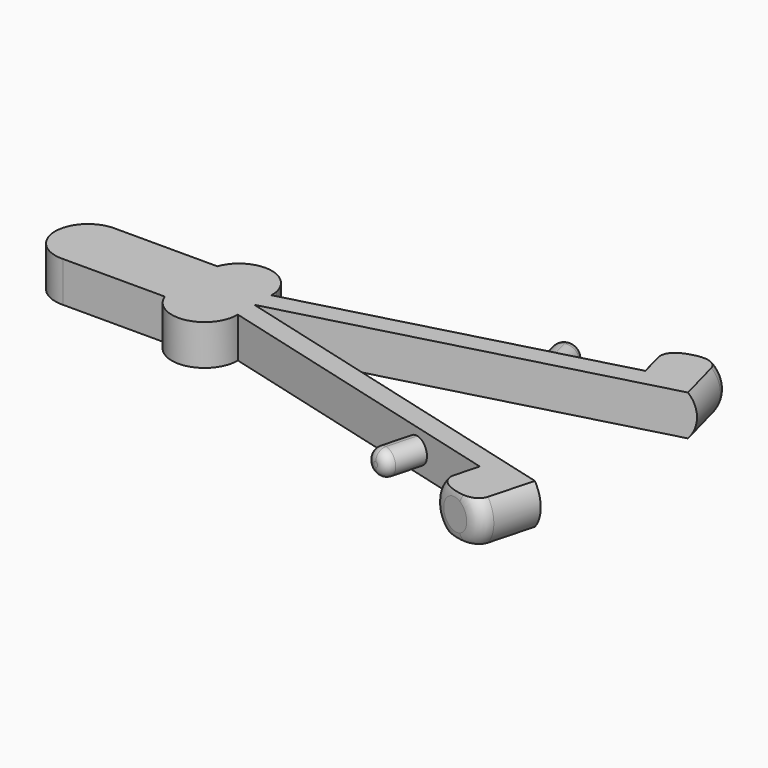
from build123d import *

# Parameters (mm, degrees)
F1_DEPTH    = 8
F4_DEPTH    = 12
F5_DEPTH    = 12
F6_DEPTH    = 4
F7_T2_ANGLE = 226.9097490639
F7_T4_ANGLE = 226.9097490639
F8_R        = 2


# Not quite as in the source:
# - a fillet or chamfer that OpenCascade refuses, or shapes differently, is made with other operations: its cross-section is extruded or revolved along the edge and cut away or added
# - a feature names something its author has since deleted; it is built from what else it names


with BuildPart() as f1:
    # F0 (on Top) → F1 (new body)
    with BuildSketch(Plane.XY):
        with BuildLine():
            ThreePointArc((-26.2934756426, -6.4967182246), (-21.8313594954, -4.5225872947), (-20, 0))
            ThreePointArc((-20, 0), (-21.8313594954, 4.5225872947), (-26.2934756426, 6.4967182246))
            ThreePointArc((-26.2934756426, 6.4967182246), (-33, 0), (-26.2934756426, -6.4967182246))
        make_face()
        with BuildLine():
            ThreePointArc((4.9180788932, 0), (0, 2.25), (-4.9180788932, 0))
            ThreePointArc((-4.9180788932, 0), (0, -2.25), (4.9180788932, 0))
        make_face()
        with BuildLine():
            Line((6.4380174247, 0), (6.3926786471, 3.0737093407))
            ThreePointArc((6.3926786471, 3.0737093407), (5.8604804677, 1.4384579519), (4.9180788932, 0))
            ThreePointArc((4.9180788932, 0), (6.0748085227, -1.9377064606), (6.4992929884, -4.1541321195))
            Line((6.4992929884, -4.1541321195), (6.4380174247, 0))
        make_face()
        with BuildLine():
            ThreePointArc((-26.2934756426, 6.4967182246), (-21.8313594954, 4.5225872947), (-20, 0))
            ThreePointArc((-20, 0), (-21.8313594954, -4.5225872947), (-26.2934756426, -6.4967182246))
            Line((-26.2934756426, -6.4967182246), (-6.0993653128, -6.4967182246))
            ThreePointArc((-6.0993653128, -6.4967182246), (-6.3951431673, -3.0871827877), (-4.9180788932, 0))
            ThreePointArc((-4.9180788932, 0), (-6.3951431673, 3.0871827877), (-6.0993653128, 6.4967182246))
            Line((-6.0993653128, 6.4967182246), (-26.2934756426, 6.4967182246))
        make_face()
        with BuildLine():
            ThreePointArc((-4.9180788932, 0), (-6.3951431673, -3.0871827877), (-6.0993653128, -6.4967182246))
            ThreePointArc((-6.0993653128, -6.4967182246), (1.141079635, -10.6490575296), (6.5, -4.25))
            ThreePointArc((6.5, -4.25), (6.4998232447, -4.2020647563), (6.4992929884, -4.1541321195))
            ThreePointArc((6.4992929884, -4.1541321195), (6.0748085227, -1.9377064606), (4.9180788932, 0))
            ThreePointArc((4.9180788932, 0), (0, -2.25), (-4.9180788932, 0))
        make_face()
        with BuildLine():
            ThreePointArc((6.3552032224, 5.614328407), (0.4593650036, 10.7337476658), (-6.0993653128, 6.4967182246))
            ThreePointArc((-6.0993653128, 6.4967182246), (-6.3951431673, 3.0871827877), (-4.9180788932, 0))
            ThreePointArc((-4.9180788932, 0), (0, 2.25), (4.9180788932, 0))
            ThreePointArc((4.9180788932, 0), (5.8604804677, 1.4384579519), (6.3926786471, 3.0737093407))
            Line((6.3926786471, 3.0737093407), (6.3552032224, 5.614328407))
        make_face()
        with BuildLine():
            ThreePointArc((6.5, 4.25), (6.4636994417, 4.9359952822), (6.3552032224, 5.614328407))
            Line((6.3552032224, 5.614328407), (6.3926786471, 3.0737093407))
            ThreePointArc((6.3926786471, 3.0737093407), (6.4731140576, 3.6594118212), (6.5, 4.25))
        make_face()
    extrude(amount=F1_DEPTH)



with BuildPart() as f4:
    # F3 (on line) → F4 (new body)
    with BuildSketch(Plane(origin=(0.4312653925, -1.6095043562, 0), x_dir=(-0.9659258263, -0.2588190451, 0), z_dir=(-0.2588190451, 0.9659258263, 0))):
        with BuildLine():
            Line((-79.4407832557, 0), (-74.9686473007, 0))
            Line((-74.9686473007, 0), (-74.9686473007, 8))
            Line((-74.9686473007, 8), (-79.4407832557, 8))
            ThreePointArc((-79.4407832557, 8), (-80.9686473007, 4), (-79.4407832557, 0))
        make_face()
        with BuildLine():
            Line((-74.9686473007, 8), (-74.9686473007, 0))
            Line((-74.9686473007, 0), (-70.4965113457, 0))
            ThreePointArc((-70.4965113457, 0), (-69.3636131469, 1.8590674614), (-68.9686473007, 4))
            ThreePointArc((-68.9686473007, 4), (-69.3636131469, 6.1409325386), (-70.4965113457, 8))
            Line((-70.4965113457, 8), (-74.9686473007, 8))
        make_face()
    extrude(amount=F4_DEPTH)


with BuildPart() as f5:
    # F3 (on line) → F5 (new body)
    with BuildSketch(Plane(origin=(0.4312653925, -1.6095043562, 0), x_dir=(-0.9659258263, -0.2588190451, 0), z_dir=(-0.2588190451, 0.9659258263, 0))):
        with BuildLine():
            ThreePointArc((-54.2186473007, 6.5), (-56.7186473007, 4), (-54.2186473007, 1.5))
            Line((-54.2186473007, 1.5), (-54.2186473007, 4))
            Line((-54.2186473007, 4), (-54.2186473007, 6.5))
        make_face()
        with BuildLine():
            ThreePointArc((-51.7186473007, 4), (-52.4508803477, 5.767766953), (-54.2186473007, 6.5))
            Line((-54.2186473007, 6.5), (-54.2186473007, 4))
            Line((-54.2186473007, 4), (-51.7186473007, 4))
        make_face()
        with BuildLine():
            Line((-54.2186473007, 4), (-54.2186473007, 1.5))
            ThreePointArc((-54.2186473007, 1.5), (-52.4508803477, 2.232233047), (-51.7186473007, 4))
            Line((-51.7186473007, 4), (-54.2186473007, 4))
        make_face()
    extrude(amount=F5_DEPTH)


with BuildPart() as f1_1:
    add(f1.part)

    add(f4.part)  # F6 merges F4

    add(f5.part)  # F6 merges F5
    # F3 (on line) → F6 (join)
    with BuildSketch(Plane(origin=(0.4312653925, -1.6095043562, 0), x_dir=(-0.9659258263, -0.2588190451, 0), z_dir=(-0.2588190451, 0.9659258263, 0))):
        with BuildLine():
            Line((-54.2186473007, 1.5), (-54.2186473007, 0))
            Line((-54.2186473007, 0), (-6.2186473007, 0))
            Line((-6.2186473007, 0), (-6.2186473007, 4))
            Line((-6.2186473007, 4), (-51.7186473007, 4))
            ThreePointArc((-51.7186473007, 4), (-52.4508803477, 2.232233047), (-54.2186473007, 1.5))
        make_face()
        with BuildLine():
            Line((-6.2186473007, 8), (-54.2186473007, 8))
            Line((-54.2186473007, 8), (-54.2186473007, 6.5))
            ThreePointArc((-54.2186473007, 6.5), (-52.4508803477, 5.767766953), (-51.7186473007, 4))
            Line((-51.7186473007, 4), (-6.2186473007, 4))
            Line((-6.2186473007, 4), (-6.2186473007, 8))
        make_face()
        with BuildLine():
            ThreePointArc((-68.9686473007, 4), (-69.3636131469, 1.8590674614), (-70.4965113457, 0))
            Line((-70.4965113457, 0), (-54.2186473007, 0))
            Line((-54.2186473007, 0), (-54.2186473007, 1.5))
            ThreePointArc((-54.2186473007, 1.5), (-56.7186473007, 4), (-54.2186473007, 6.5))
            Line((-54.2186473007, 6.5), (-54.2186473007, 8))
            Line((-54.2186473007, 8), (-70.4965113457, 8))
            ThreePointArc((-70.4965113457, 8), (-69.3636131469, 6.1409325386), (-68.9686473007, 4))
        make_face()
    extrude(amount=F6_DEPTH)

    # F7: fillet of radius 3 on 2 edges, made by hand

    # F7_s1 → F7_t2 (revolve, cut)
    with BuildSketch(Plane(origin=(62.3527130216, 16.7073591, 28.0076976241), x_dir=(-0.2588190451, 0.9659258263, 0), z_dir=(0.8861150843, 0.2374338212, 0.3980266798))):
        with BuildLine():
            ThreePointArc((7.3337184778, -32.1700264164), (9.4550388213, -31.2913467599), (10.3337184778, -29.1700264164))
            Line((10.3337184778, -29.1700264164), (10.3337184778, -32.1700264164))
            Line((10.3337184778, -32.1700264164), (7.3337184778, -32.1700264164))
        make_face()
    revolve(axis=Axis((69.7395894409, 29.3849192663, 4), (-0.2588190451, 0.9659258263, 0)), revolution_arc=F7_T2_ANGLE, mode=Mode.SUBTRACT)

    # F7_s3 → F7_t4 (revolve, cut)
    with BuildSketch(Plane(origin=(62.3527130216, 16.7073591, 28.0076976241), x_dir=(0.2588190451, -0.9659258263, 0), z_dir=(-0.8861150843, -0.2374338212, -0.3980266798))):
        with BuildLine():
            ThreePointArc((-7.3337184778, -20.1700264164), (-9.4550388213, -21.0487060728), (-10.3337184778, -23.1700264164))
            Line((-10.3337184778, -23.1700264164), (-10.3337184778, -20.1700264164))
            Line((-10.3337184778, -20.1700264164), (-7.3337184778, -20.1700264164))
        make_face()
    revolve(axis=Axis((69.7395894409, 29.3849192663, 4), (-0.2588190451, 0.9659258263, 0)), revolution_arc=F7_T4_ANGLE, mode=Mode.SUBTRACT)

    # F8
    f8_edges = [f1_1.edges().sort_by_distance(p)[0] for p in [
        (49.696629, 24.014424, 6.5),
    ]]
    fillet(f8_edges, radius=F8_R)

    # F9: F1 across plane


with BuildPart() as f1_2:
    add(f1_1.part)
    add(f1_1.part.mirror(Plane.XZ))


solid = f1_2.part
